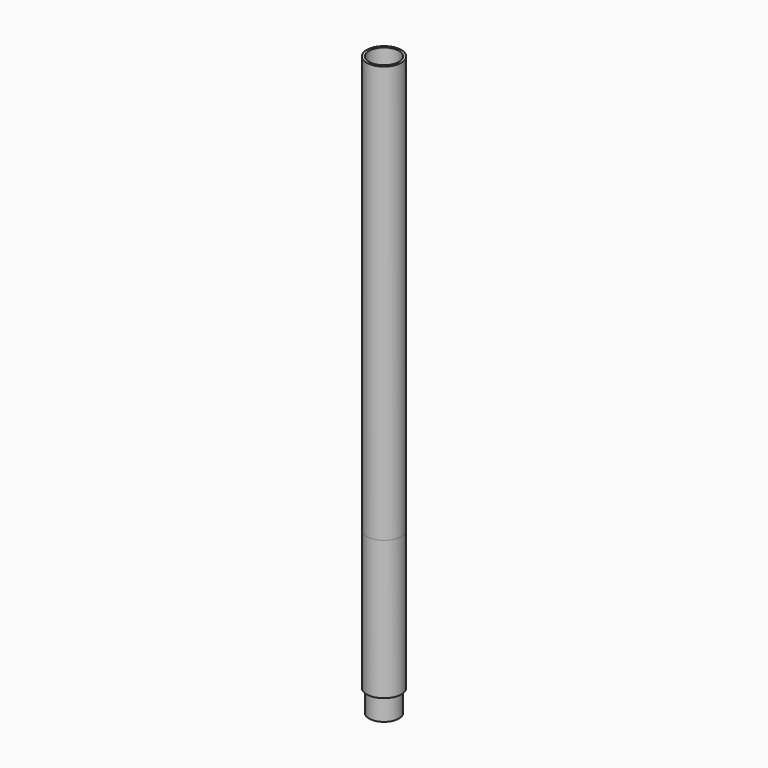
from build123d import *

# Parameters (mm, degrees)
F0_R     = 25
F0_R_2   = 21.5
F1_DEPTH = 800
F2_DEPTH = 200
F3_W     = 30
F3_H     = 30
F4_DEPTH = 25.001


with BuildPart() as f1:
    # F0 (on Top) → F1 (new body)
    with BuildSketch(Plane.XY):
        Circle(F0_R)
        Circle(F0_R_2, mode=Mode.SUBTRACT)
    extrude(amount=F1_DEPTH)


with BuildPart() as f2:
    # F0 (on Top) → F2 (new body)
    with BuildSketch(Plane.XY):
        Circle(F0_R)
        Circle(F0_R_2, mode=Mode.SUBTRACT)
    extrude(amount=F2_DEPTH)

    # F3 (on Right) → F4 (cut, through all)
    with BuildSketch(Plane.YZ):
        with Locations((0, 95)):
            Rectangle(F3_W, F3_H)
    extrude(amount=-F4_DEPTH, mode=Mode.SUBTRACT)

    # F5 (on Front) → F6 (revolve)
    with BuildSketch(Plane.XZ):
        Polygon((-16.5, -31.8300328033), (-16.5, 0), (-16.5, 28.1699671967), (-21.5, 28.1699671967), (-21.5, -31.8300328033), align=None)
    revolve(axis=Axis((0, 0, -0.3124903888), (0, 0, -1)))


solid = Compound([f1.part, f2.part])
